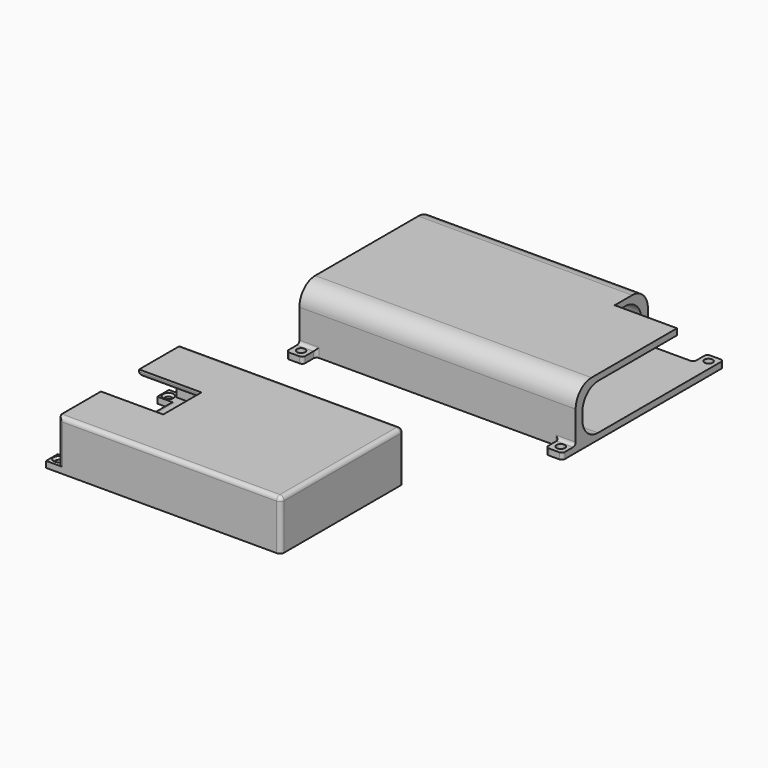
from build123d import *

# Parameters (mm, degrees)
F1_DEPTH  = 25
F0_W      = 8
F0_H      = 8
F0_R      = 2
F0_W_2    = 26
F0_H_2    = 16
F0_W_3    = 4
F0_H_3    = 57
F2_DEPTH  = 3
F3_START  = 25
F3_DEPTH  = 3
F4_R      = 1.5
F5_R      = 9.5
F6_R      = 1.55
F7_DEPTH  = 3
F8_DEPTH  = 21
F9_START  = 21
F9_DEPTH  = 3
F10_W     = 30
F10_H     = 23
F11_DEPTH = 3
F12_R     = 2
F13_SIZE  = 1


with BuildPart() as f1:
    # F0 (on Top) → F1 (new body)
    with BuildSketch(Plane.XY):
        Polygon((-60.0788152814, -9.3025659323), (-60.0788152814, 63.6974340677), (38.9211847186, 63.6974340677), (38.9211847186, 67.6974340677), (-56.0788152814, 67.6974340677), (-64.0788152814, 67.6974340677), (-64.0788152814, -13.3025659323), (-56.0788152814, -13.3025659323), (60.9211847186, -13.3025659323), (68.9211847186, -13.3025659323), (68.9211847186, -9.3025659323), (64.9211847186, -9.3025659323), align=None)
    extrude(amount=F1_DEPTH)

    # F0 (on Top) → F2 (join)
    with BuildSketch(Plane.XY):
        with Locations((-60.0788152814, 71.6974340677)):
            Rectangle(F0_W, F0_H)
        with Locations((-60.0788152814, 71.6974340677)):
            Circle(F0_R, mode=Mode.SUBTRACT)
        with Locations((64.9211847186, 71.6974340677)):
            Rectangle(F0_W, F0_H)
        with Locations((64.9211847186, 71.6974340677)):
            Circle(F0_R, mode=Mode.SUBTRACT)
        Polygon((38.9211847186, 67.6974340677), (38.9211847186, 63.6974340677), (64.9211847186, 63.6974340677), (68.9211847186, 63.6974340677), (68.9211847186, 67.6974340677), (60.9211847186, 67.6974340677), align=None)
        with Locations((51.9211847186, 55.6974340677)):
            Rectangle(F0_W_2, F0_H_2)
        with Locations((66.9211847186, 55.6974340677)):
            Rectangle(F0_W_3, F0_H_2)
        with Locations((66.9211847186, 19.1974340677)):
            Rectangle(F0_W_3, F0_H_3)
        Polygon((38.9211847186, 63.6974340677), (-60.0788152814, 63.6974340677), (-60.0788152814, -9.3025659323), (64.9211847186, -9.3025659323), (64.9211847186, 47.6974340677), (38.9211847186, 47.6974340677), align=None)
        with Locations((64.9211847186, -17.3025659323)):
            Rectangle(F0_W, F0_H)
        with Locations((64.9211847186, -17.3025659323)):
            Circle(F0_R, mode=Mode.SUBTRACT)
        with Locations((-60.0788152814, -17.3025659323)):
            Rectangle(F0_W, F0_H)
        with Locations((-60.0788152814, -17.3025659323)):
            Circle(F0_R, mode=Mode.SUBTRACT)
    extrude(amount=F2_DEPTH)

    # F0 (on Top) → F3 (join)
    with BuildSketch(Plane.XY.offset(F3_START)):
        Polygon((-60.0788152814, -9.3025659323), (-60.0788152814, 63.6974340677), (38.9211847186, 63.6974340677), (38.9211847186, 67.6974340677), (-56.0788152814, 67.6974340677), (-64.0788152814, 67.6974340677), (-64.0788152814, -13.3025659323), (-56.0788152814, -13.3025659323), (60.9211847186, -13.3025659323), (68.9211847186, -13.3025659323), (68.9211847186, -9.3025659323), (64.9211847186, -9.3025659323), align=None)
        Polygon((38.9211847186, 63.6974340677), (-60.0788152814, 63.6974340677), (-60.0788152814, -9.3025659323), (64.9211847186, -9.3025659323), (64.9211847186, 47.6974340677), (38.9211847186, 47.6974340677), align=None)
        with Locations((66.9211847186, 19.1974340677)):
            Rectangle(F0_W_3, F0_H_3)
    extrude(amount=F3_DEPTH)

    # F4
    f4_edges = [f1.edges().sort_by_distance(p)[0] for p in [
        (64.921185, -13.302566, 3),
        (-60.078815, -13.302566, 3),
        (-60.078815, 67.697434, 3),
        (60.921185, 67.697434, 1.5),
        (-56.078815, 67.697434, 1.5),
        (-56.078815, -13.302566, 1.5),
        (60.921185, -13.302566, 1.5),
        (38.921185, 65.697434, 3),
        (-56.078815, 75.697434, 1.5),
        (-56.078815, -21.302566, 1.5),
        (-64.078815, -21.302566, 1.5),
        (60.921185, -21.302566, 1.5),
        (68.921185, -21.302566, 1.5),
        (68.921185, 75.697434, 1.5),
        (60.921185, 75.697434, 1.5),
    ]]
    fillet(f4_edges, radius=F4_R)

    # F5
    f5_edges = [f1.edges().sort_by_distance(p)[0] for p in [
        (-10.578815, 63.697434, 25),
        (-10.578815, 63.697434, 3),
        (4.421185, -9.302566, 3),
        (4.421185, -9.302566, 25),
        (2.421185, -13.302566, 28),
        (-12.578815, 67.697434, 28),
    ]]
    fillet(f5_edges, radius=F5_R)


with BuildPart() as f7:
    # F6 (on Top) → F7 (new body)
    with BuildSketch(Plane.XY):
        Polygon((31.1341558844, -76.2936508735), (-72.8658441156, -76.2936508735), (-72.8658441156, -80.2936508735), (-72.8658441156, -140.2936508735), (-72.8658441156, -144.2936508735), (31.1341558844, -144.2936508735), align=None)
        Polygon((-72.8658441156, -73.2936508735), (-72.8658441156, -76.2936508735), (31.1341558844, -76.2936508735), (31.1341558844, -144.2936508735), (-72.8658441156, -144.2936508735), (-72.8658441156, -147.2936508735), (34.1341558844, -147.2936508735), (34.1341558844, -73.2936508735), align=None)
        Polygon((-72.8658441156, -80.2936508735), (-72.8658441156, -76.2936508735), (-72.8658441156, -73.2936508735), (-78.8658441156, -73.2936508735), (-78.8658441156, -80.2936508735), align=None)
        with Locations((-75.9158441156, -77.3436508735)):
            Circle(F6_R, mode=Mode.SUBTRACT)
        Polygon((-72.8658441156, -144.2936508735), (-72.8658441156, -140.2936508735), (-78.8658441156, -140.2936508735), (-78.8658441156, -147.2936508735), (-72.8658441156, -147.2936508735), align=None)
        with Locations((-75.9158441156, -143.2436508735)):
            Circle(F6_R, mode=Mode.SUBTRACT)
    extrude(amount=F7_DEPTH)

    # F6 (on Top) → F8 (join)
    with BuildSketch(Plane.XY):
        Polygon((-72.8658441156, -73.2936508735), (-72.8658441156, -76.2936508735), (31.1341558844, -76.2936508735), (31.1341558844, -144.2936508735), (-72.8658441156, -144.2936508735), (-72.8658441156, -147.2936508735), (34.1341558844, -147.2936508735), (34.1341558844, -73.2936508735), align=None)
    extrude(amount=F8_DEPTH)

    # F6 (on Top) → F9 (join)
    with BuildSketch(Plane.XY.offset(F9_START)):
        Polygon((-72.8658441156, -73.2936508735), (-72.8658441156, -76.2936508735), (31.1341558844, -76.2936508735), (31.1341558844, -144.2936508735), (-72.8658441156, -144.2936508735), (-72.8658441156, -147.2936508735), (34.1341558844, -147.2936508735), (34.1341558844, -73.2936508735), align=None)
        Polygon((31.1341558844, -76.2936508735), (-72.8658441156, -76.2936508735), (-72.8658441156, -80.2936508735), (-72.8658441156, -140.2936508735), (-72.8658441156, -144.2936508735), (31.1341558844, -144.2936508735), align=None)
    extrude(amount=F9_DEPTH)

    # F10 (on face) → F11 (cut)
    with BuildSketch(Plane.XY.offset(24)):
        with Locations((-57.8658441156, -110.2936508735)):
            Rectangle(F10_W, F10_H)
    extrude(amount=-F11_DEPTH, mode=Mode.SUBTRACT)

    # F12
    f12_edges = [f7.edges().sort_by_distance(p)[0] for p in [
        (-19.365844, -73.293651, 24),
        (-19.365844, -147.293651, 24),
        (34.134156, -110.293651, 24),
        (34.134156, -147.293651, 12),
        (34.134156, -73.293651, 12),
        (-72.865844, -147.293651, 13.5),
        (-72.865844, -73.293651, 13.5),
        (-72.865844, -133.043651, 21),
        (-72.865844, -87.543651, 21),
        (-57.865844, -98.793651, 21),
        (-57.865844, -121.793651, 21),
        (-42.865844, -110.293651, 21),
        (-72.865844, -110.293651, 3),
    ]]
    fillet(f12_edges, radius=F12_R)

    # F13
    f13_edges = [f7.edges().sort_by_distance(p)[0] for p in [
        (-77.465844, -77.343651, 3),
        (-77.465844, -143.243651, 3),
    ]]
    chamfer(f13_edges, length=F13_SIZE)


solid = Compound([f1.part, f7.part])
